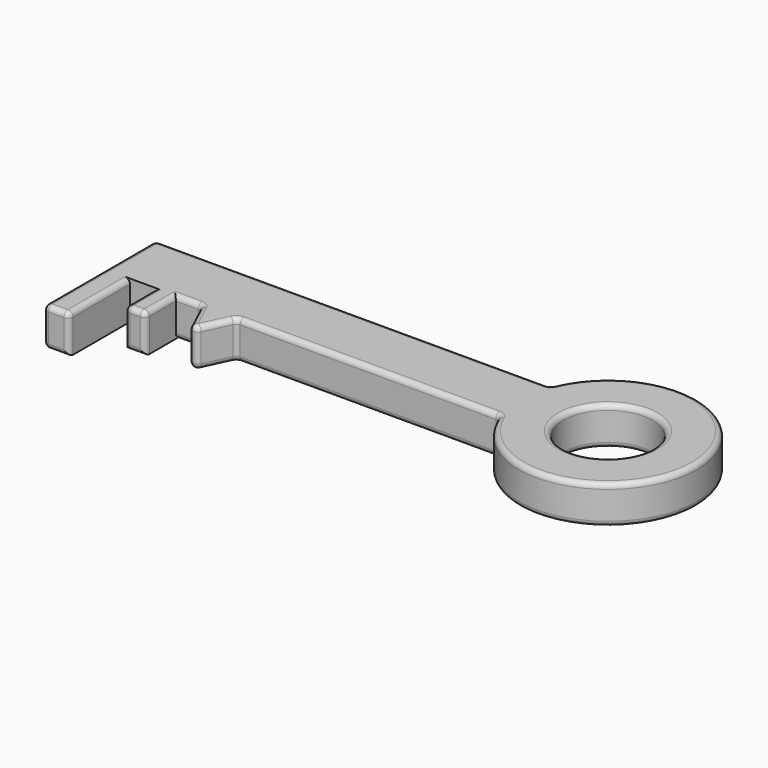
from build123d import *

# Parameters (mm, degrees)
F0_W     = 10
F0_H     = 30
F0_W_2   = 8
F0_H_2   = 15
F0_R     = 17.5
F1_DEPTH = 15
F2_R     = 2


with BuildPart() as f1:
    # F0 (on Top) → F1 (new body)
    with BuildSketch(Plane.XY):
        with Locations((-150, -4.3002969027)):
            Rectangle(F0_W, F0_H)
        with Locations((-131, 3.1997030973)):
            Rectangle(F0_W_2, F0_H_2)
        Polygon((-109.9998707869, -4.3002969027), (-102.9997415738, 10.6997030973), (-117, 10.6997030973), align=None)
        with BuildLine():
            Line((0, 35.6997030973), (0, 10.6997030973))
            ThreePointArc((0, 10.6997030973), (67.6917420766, 23.1997030973), (0, 35.6997030973))
        make_face()
        with Locations((32.6917420766, 23.1997030973)):
            Circle(F0_R, mode=Mode.SUBTRACT)
        Polygon((-102.9997415738, 10.6997030973), (0, 10.6997030973), (0, 35.6997030973), (-155, 35.6997030973), (-155, 10.6997030973), (-145, 10.6997030973), (-135, 10.6997030973), (-127, 10.6997030973), (-117, 10.6997030973), align=None)
    extrude(amount=F1_DEPTH)

    # F2
    f2_edges = [f1.edges().sort_by_distance(p)[0] for p in [
        (-77.5, 35.699703, 15),
        (67.691742, 23.199703, 15),
        (15.191742, 23.199703, 15),
        (-51.499871, 10.699703, 15),
        (-106.499806, 3.199703, 15),
        (-113.499935, 3.199703, 15),
        (-127, 3.199703, 15),
        (-131, -4.300297, 15),
        (-135, 3.199703, 15),
        (-145, -4.300297, 15),
        (-150, -19.300297, 15),
        (-155, 8.199703, 15),
        (-77.5, 35.699703, 0),
        (67.691742, 23.199703, 0),
        (15.191742, 23.199703, 0),
        (-102.999742, 10.699703, 7.5),
        (-109.999871, -4.300297, 7.5),
        (-117, 10.699703, 7.5),
        (-127, -4.300297, 7.5),
        (-145, -19.300297, 7.5),
        (-135, -4.300297, 7.5),
        (-155, -19.300297, 7.5),
        (0, 10.699703, 7.5),
        (-51.499871, 10.699703, 0),
        (-106.499806, 3.199703, 0),
        (-113.499935, 3.199703, 0),
        (-131, -4.300297, 0),
        (-150, -19.300297, 0),
        (-122, 10.699703, 0),
        (-140, 10.699703, 0),
        (-155, 8.199703, 0),
        (-155, 35.699703, 7.5),
        (0, 35.699703, 7.5),
        (-122, 10.699703, 15),
    ]]
    fillet(f2_edges, radius=F2_R)


solid = f1.part
